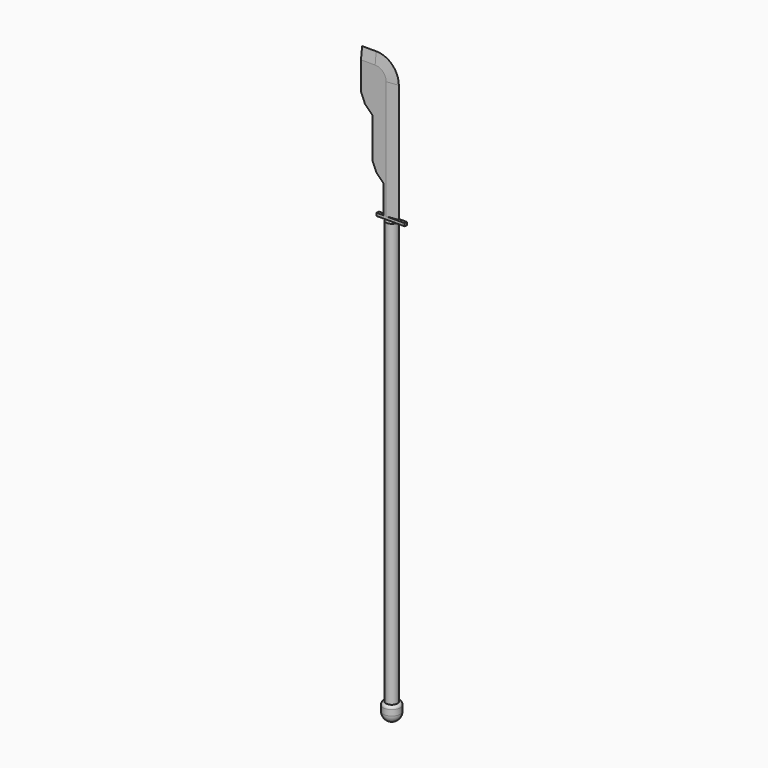
from build123d import *

# Parameters (mm, degrees)
F0_R          = 25.4
F1_DEPTH      = 1905
F2_R          = 38.1
F3_DEPTH      = 76.2
F4_W          = 50.8
F4_H          = 254
F5_DEPTH      = 6.35
F5_DEPTH_BACK = 6.35
F6_SIZE       = 50.79999
F7_R          = 101.6
F8_SIZE2      = 51.71659
F8_SIZE       = 6.34999
F9_SIZE       = 25.4
F11_R         = 38.1


# Not quite as in the source:
# - a fillet or chamfer that OpenCascade refuses, or shapes differently, is made with other operations: its cross-section is extruded or revolved along the edge and cut away or added
# - a fillet or chamfer is up to 0.001 mm smaller than in the source, because OpenCascade refuses the exact size


with BuildPart() as f1:
    # F0 (on Top) → F1 (new body)
    with BuildSketch(Plane.XY):
        Circle(F0_R)
    extrude(amount=F1_DEPTH)

    # F2 (on face) → F3 (join)
    with BuildSketch(Plane(origin=(0, 0, 0), x_dir=(1, 0, 0), z_dir=(0, 0, -1))):
        Circle(F2_R)
    extrude(amount=F3_DEPTH)

    # F4 (on Front) → F5 (join, two sides)
    with BuildSketch(Plane.XZ) as f5_sk:
        Polygon((-25.4, 1905), (0, 1905), (25.4, 1905), (63.5, 1905), (63.5, 1917.7), (31.75, 1917.7), (0, 1917.7), (-31.75, 1917.7), (-63.5, 1917.7), (-63.5, 1905), align=None)
        Polygon((0, 1917.7), (31.75, 1917.7), (31.75, 2552.7), (-31.75, 2552.7), (-31.75, 2298.7), (-31.75, 2044.7), (-31.75, 1917.7), align=None)
        with Locations((-57.15, 2171.7)):
            Rectangle(F4_W, F4_H)
        Polygon((-31.75, 2298.7), (-31.75, 2552.7), (-133.35, 2552.7), (-133.35, 2298.7), (-82.55, 2298.7), align=None)
    extrude(amount=F5_DEPTH)
    extrude(f5_sk.sketch, amount=-F5_DEPTH_BACK)

    # F6 (size 50.8 in the source; OpenCascade refuses exactly that, so slightly less here)
    f6_edges = [f1.edges().sort_by_distance(p)[0] for p in [
        (-133.35, 0, 2298.7),
        (-82.55, 0, 2044.7),
    ]]
    chamfer(f6_edges, length=F6_SIZE)

    # F7
    f7_edges = [f1.edges().sort_by_distance(p)[0] for p in [
        (31.75, 0, 2552.7),
    ]]
    fillet(f7_edges, radius=F7_R)

    # F8 (size 6.35 and 51.7165998176 in the source; OpenCascade refuses exactly that, so slightly less here)
    f8_edges = [f1.edges().sort_by_distance(p)[0] for p in [
        (31.75, 6.35, 2184.4),
        (31.75, -6.35, 2184.4),
    ]]
    f8_side = f1.faces().sort_by_distance((31.75, 0, 2184.4))[0]
    chamfer(f8_edges, length=F8_SIZE, length2=F8_SIZE2, reference=f8_side)

    # F9
    f9_edges = [f1.edges().sort_by_distance(p)[0] for p in [
        (-133.35, 0, 2349.49999),
        (-82.55, 0, 2095.49999),
    ]]
    chamfer(f9_edges, length=F9_SIZE)

    # F10: fillet of radius 12.7 on 1 edges, made by hand

    # F10_s1 → F10_t2 (revolve, cut)
    with BuildSketch(Plane.XZ):
        with BuildLine():
            ThreePointArc((25.4, 0), (34.3802561211, -3.7197438789), (38.1, -12.7))
            Line((38.1, -12.7), (38.1, 0))
            Line((38.1, 0), (25.4, 0))
        make_face()
    revolve(axis=Axis((0, 0, 0), (0, 0, -1)), mode=Mode.SUBTRACT)

    # F11
    f11_edges = [f1.edges().sort_by_distance(p)[0] for p in [
        (-38.1, 0, -76.2),
    ]]
    fillet(f11_edges, radius=F11_R)


solid = f1.part
